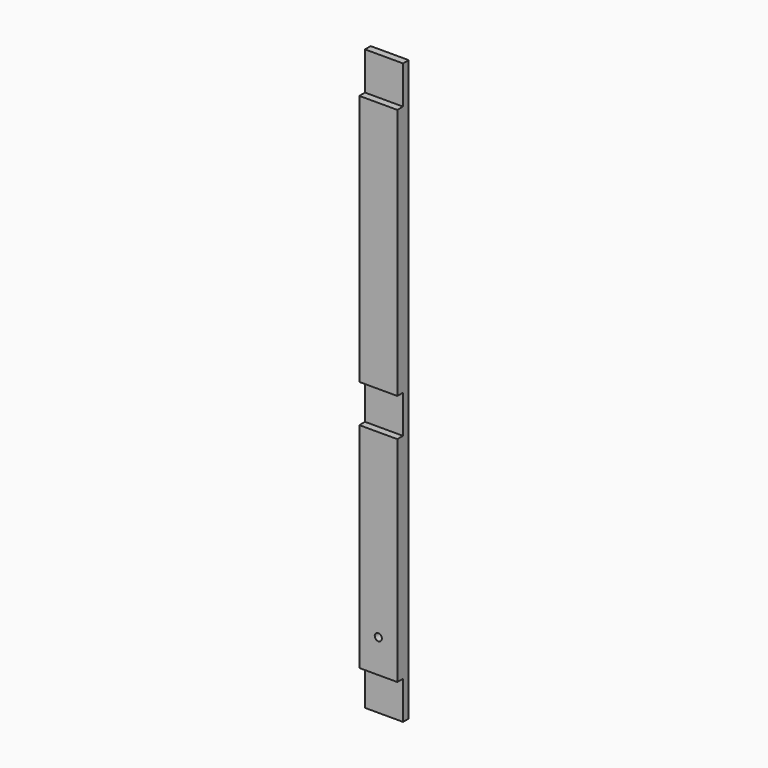
from build123d import *

# Parameters (mm, degrees)
F0_W     = 50.8
F0_H     = 19.05
F1_DEPTH = 774.7
F2_W     = 122.43557321
F2_H     = 50.8
F2_W_2   = 343.1604206562
F2_W_3   = 264.5317912102
F3_DEPTH = 25.4
F4_R     = 0.79375
F5_DEPTH = 25.4
F6_R     = 4.7625
F7_DEPTH = 25.4


# Not quite as in the source:
# - a feature names something its author has since deleted; it is built from what else it names


with BuildPart() as f1:
    # F0 (on Top) → F1 (new body)
    with BuildSketch(Plane.XY):
        Rectangle(F0_W, F0_H)
    extrude(amount=F1_DEPTH)

    # F2 (on Front) → F3 (cut)
    with BuildSketch(Plane.XZ):
        with Locations((22.4465244144, 25.4)):
            Rectangle(F2_W, F2_H)
        with Locations((-38.7818217278, 749.3)):
            Rectangle(F2_W_2, F2_H)
        with Locations((-47.6498156786, 361.95)):
            Rectangle(F2_W_3, F2_H)
    extrude(amount=F3_DEPTH, mode=Mode.SUBTRACT)

    # F4 (on Front) → F5 (cut)
    with BuildSketch(Plane.XZ):
        with Locations((9.525, 101.6)):
            Circle(F4_R)
        with Locations((9.525, 155.575)):
            Circle(F4_R)
        with Locations((9.525, 619.125)):
            Circle(F4_R)
        with Locations((9.525, 673.1)):
            Circle(F4_R)
        with Locations((-9.525, 619.125)):
            Circle(F4_R)
        with Locations((-9.525, 673.1)):
            Circle(F4_R)
        with Locations((-9.525, 101.6)):
            Circle(F4_R)
        with Locations((-9.525, 155.575)):
            Circle(F4_R)
    extrude(amount=-F5_DEPTH, mode=Mode.SUBTRACT)

    # F6 (on Front) → F7 (cut)
    with BuildSketch(Plane.XZ):
        with Locations((0, 95.25)):
            Circle(F6_R)
    extrude(amount=F7_DEPTH, mode=Mode.SUBTRACT)


solid = f1.part
